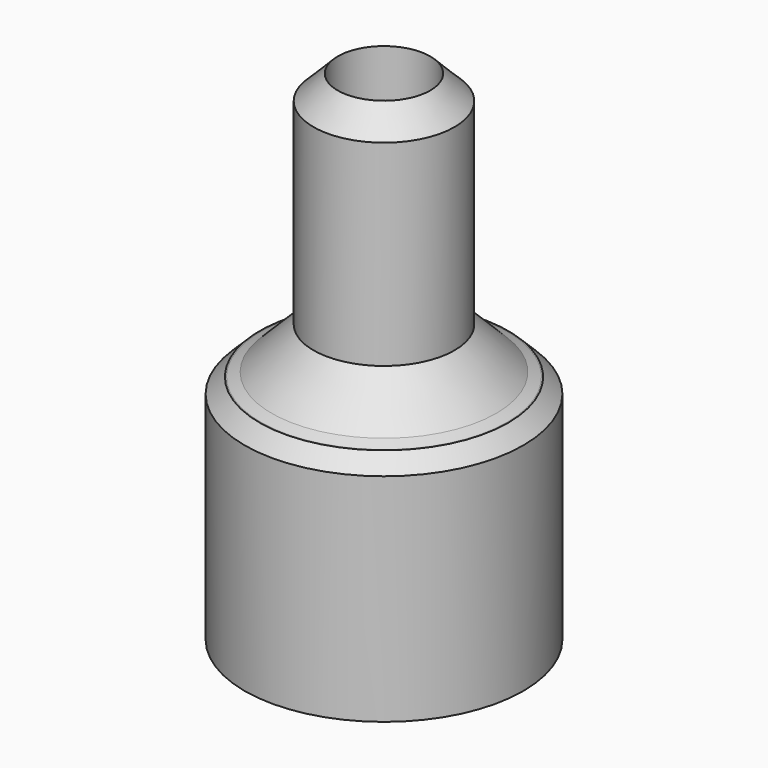
from build123d import *

# Parameters (mm, degrees)
F0_R     = 12.05
F0_R_2   = 4
F1_DEPTH = 45
F2_R     = 13.7736211886
F2_R_2   = 6.1
F3_DEPTH = 25


# Not quite as in the source:
# - a fillet or chamfer that OpenCascade refuses, or shapes differently, is made with other operations: its cross-section is extruded or revolved along the edge and cut away or added


with BuildPart() as f1:
    # F0 (on Top) → F1 (new body)
    with BuildSketch(Plane.XY):
        Circle(F0_R)
        Circle(F0_R_2, mode=Mode.SUBTRACT)
    extrude(amount=F1_DEPTH)

    # F2 (on face) → F3 (cut)
    with BuildSketch(Plane.XY.offset(45)):
        Circle(F2_R)
        Circle(F2_R_2, mode=Mode.SUBTRACT)
    extrude(amount=-F3_DEPTH, mode=Mode.SUBTRACT)

    # F4: chamfer of 4 on 3 edges, made by hand

    # F4_s1 → F4_t2 (revolve)
    with BuildSketch(Plane.XZ):
        Polygon((10.1, 20), (6.1, 24), (6.1, 20), align=None)
    revolve(axis=Axis((0, 0, 20), (0, 0, 1)))

    # F4_s3 → F4_t4 (revolve, cut)
    with BuildSketch(Plane.XZ):
        Polygon((2.1, 45), (6.1, 41), (6.1, 45), align=None)
    revolve(axis=Axis((0, 0, 45), (0, 0, 1)), mode=Mode.SUBTRACT)

    # F5: chamfer of 1.3 on 2 edges, made by hand

    # F5_s1 → F5_t2 (revolve)
    with BuildSketch(Plane.XZ):
        Polygon((10.6384776311, 20), (9.7192388155, 20.3807611845), (10.1, 20), align=None)
    revolve(axis=Axis((0, 0, 20), (0, 0, 1)))

    # F5_s3 → F5_t4 (revolve, cut)
    with BuildSketch(Plane.XZ):
        Polygon((12.05, 18.7), (10.75, 20), (12.05, 20), align=None)
    revolve(axis=Axis((0, 0, 20), (0, 0, -1)), mode=Mode.SUBTRACT)


solid = f1.part
